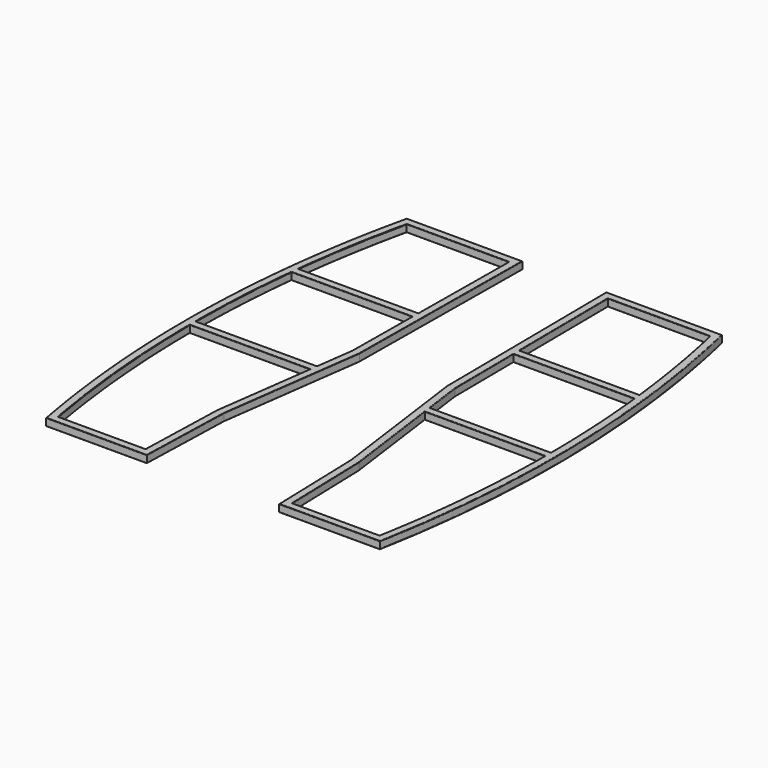
from build123d import *


with BuildPart() as f5:
    # F5: sweep along a path in F2
    with BuildLine(Plane(origin=(0, 0, -679.45), x_dir=(1, 0, 0), z_dir=(0, 0, -1))) as f5_path:
        Line((-536.575, -12.7), (-142.875, -12.7))
        Line((-142.875, -12.7), (-149.225, 673.1))
        Line((-149.225, 673.1), (-215.782412, 1165.368452))
        Line((-215.782412, 1165.368452), (-225.307412, 1482.725544))
        Line((-225.307412, 1482.725544), (-568.207412, 1482.725544))
        ThreePointArc((-568.207412, 1482.725544), (-629.170577, 733.388675), (-536.575, -12.7))
    # F4 (on line) → F5 (sweep)
    with BuildSketch(Plane(origin=(-536.575, 0, 0), x_dir=(0, -1, 0), z_dir=(-1, 0, 0))):
        with BuildLine():
            ThreePointArc((-12.7, -677.8625), (-12.235032, -678.985032), (-11.1125, -679.45))
            Line((-11.1125, -679.45), (11.1125, -679.45))
            ThreePointArc((11.1125, -679.45), (12.235032, -678.985032), (12.7, -677.8625))
            Line((12.7, -677.8625), (12.7, -655.6375))
            ThreePointArc((12.7, -655.6375), (12.235032, -654.514968), (11.1125, -654.05))
            Line((11.1125, -654.05), (-11.1125, -654.05))
            ThreePointArc((-11.1125, -654.05), (-12.235032, -654.514968), (-12.7, -655.6375))
            Line((-12.7, -655.6375), (-12.7, -677.8625))
        make_face()
    sweep(path=f5_path.line, transition=Transition.RIGHT)

    # F8: sweep along a path in F2
    with BuildLine(Plane(origin=(0, 0, -679.45), x_dir=(1, 0, 0), z_dir=(0, 0, -1))) as f8_path:
        Line((-594.882513, 406.4), (-339.725, 406.4))
        Line((-339.725, 406.4), (-172.156644, 406.4))
        Line((-172.156644, 406.4), (-159.457189, 406.517588))
    # F7 (on line) → F8 (sweep)
    with BuildSketch(Plane.YZ.offset(-339.725)):
        with BuildLine():
            Line((-406.4, -679.45), (-395.2875, -679.45))
            ThreePointArc((-395.2875, -679.45), (-394.164968, -678.985032), (-393.7, -677.8625))
            Line((-393.7, -677.8625), (-393.7, -655.6375))
            ThreePointArc((-393.7, -655.6375), (-394.164968, -654.514968), (-395.2875, -654.05))
            Line((-395.2875, -654.05), (-417.5125, -654.05))
            ThreePointArc((-417.5125, -654.05), (-418.635032, -654.514968), (-419.1, -655.6375))
            Line((-419.1, -655.6375), (-419.1, -677.8625))
            ThreePointArc((-419.1, -677.8625), (-418.635032, -678.985032), (-417.5125, -679.45))
            Line((-417.5125, -679.45), (-406.4, -679.45))
        make_face()
    sweep(path=f8_path.line)

    # F9: sweep along a path in F2
    with BuildLine(Plane(origin=(0, 0, -679.45), x_dir=(1, 0, 0), z_dir=(0, 0, -1))) as f9_path:
        Line((-617.293247, 812.8), (-339.725, 812.8))
        Line((-339.725, 812.8), (-193.54392, 812.8))
        Line((-193.54392, 812.8), (-180.84392, 812.8))
    # F7 (on line) → F9 (sweep)
    with BuildSketch(Plane.YZ.offset(-339.725)):
        with BuildLine():
            Line((-812.8, -679.45), (-801.6875, -679.45))
            ThreePointArc((-801.6875, -679.45), (-800.564968, -678.985032), (-800.1, -677.8625))
            Line((-800.1, -677.8625), (-800.1, -655.6375))
            ThreePointArc((-800.1, -655.6375), (-800.564968, -654.514968), (-801.6875, -654.05))
            Line((-801.6875, -654.05), (-823.9125, -654.05))
            ThreePointArc((-823.9125, -654.05), (-825.035032, -654.514968), (-825.5, -655.6375))
            Line((-825.5, -655.6375), (-825.5, -677.8625))
            ThreePointArc((-825.5, -677.8625), (-825.035032, -678.985032), (-823.9125, -679.45))
            Line((-823.9125, -679.45), (-812.8, -679.45))
        make_face()
    sweep(path=f9_path.line)


with BuildPart() as f10_1:
    # F10: instance of F5
    add(f5.part.mirror(Plane.YZ))


solid = Compound([f5.part, f10_1.part])
